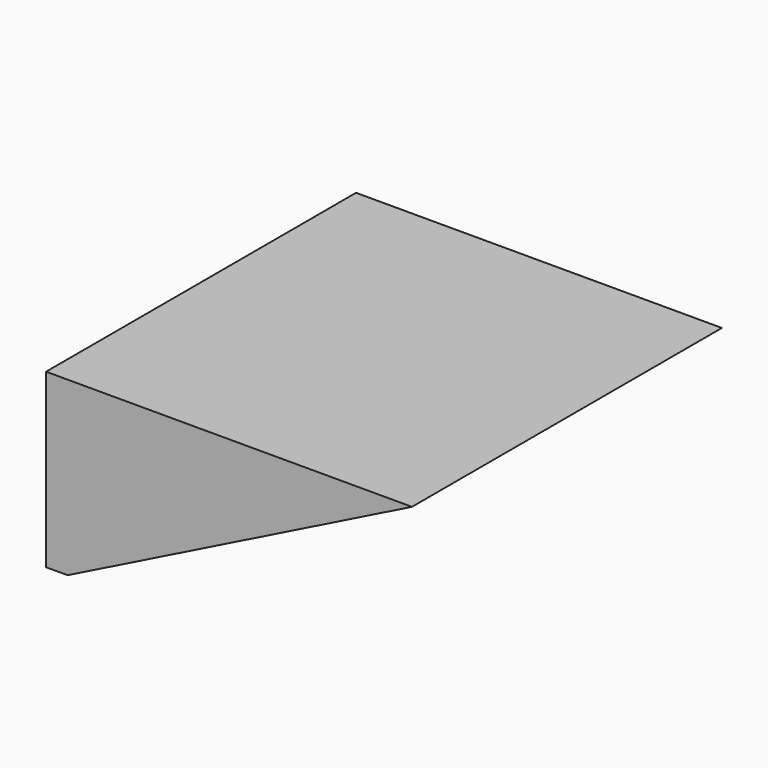
from build123d import *

# Parameters (mm, degrees)
F1_ANGLE      = 50
F3_DEPTH      = 25.4
F3_DEPTH_BACK = 25.4
F4_W          = 457.2
F4_H          = 203.2
F5_DEPTH      = 25.4
F7_DEPTH      = 406.4
F9_DEPTH      = 457.2


# Not quite as in the source:
# - ends of sketch curves that miss each other by under 0.0002 mm in the source are joined


with BuildPart() as f1:
    # F0 (on Top) → F1 (revolve)
    with BuildSketch(Plane.XY):
        with BuildLine():
            Line((-12.7, 12.7), (12.7, 12.7))
            ThreePointArc((12.7, 12.7), (0, 25.4), (-12.7, 12.7))
        make_face()
        with BuildLine():
            ThreePointArc((0, 0), (8.9802561211, 3.7197438789), (12.7, 12.7))
            Line((12.7, 12.7), (-12.7, 12.7))
            ThreePointArc((-12.7, 12.7), (-8.9802561211, 3.7197438789), (0, 0))
        make_face()
        with BuildLine():
            ThreePointArc((0, 0), (-8.9802561211, 3.7197438789), (-12.7, 12.7))
            Line((-12.7, 12.7), (-12.7, -12.7))
            ThreePointArc((-12.7, -12.7), (-8.9802561211, -3.7197438789), (0, 0))
        make_face()
        with BuildLine():
            Line((-12.7, -12.7), (12.7, -12.7))
            ThreePointArc((12.7, -12.7), (8.9802561211, -3.7197438789), (0, 0))
            ThreePointArc((0, 0), (-8.9802561211, -3.7197438789), (-12.7, -12.7))
        make_face()
        with BuildLine():
            ThreePointArc((-12.7, -12.7), (0, -25.4), (12.7, -12.7))
            Line((12.7, -12.7), (-12.7, -12.7))
        make_face()
        with BuildLine():
            Line((12.7, -12.7), (12.7, 12.7))
            ThreePointArc((12.7, 12.7), (8.9802561211, 3.7197438789), (0, 0))
            ThreePointArc((0, 0), (8.9802561211, -3.7197438789), (12.7, -12.7))
        make_face()
    revolve(axis=Axis((254, -3.8792621344, 0), (0, 1, 0)), revolution_arc=F1_ANGLE)

    # F2 (on Front) → F3 (cut, two sides)
    with BuildSketch(Plane.XZ) as f3_sk:
        Polygon((106.0351878405, 182.2580546141), (82.3100507259, 209.7299993038), (82.3100507259, 161.4786684513), align=None)
    extrude(amount=-F3_DEPTH, mode=Mode.SUBTRACT)
    extrude(f3_sk.sketch, amount=F3_DEPTH_BACK, mode=Mode.SUBTRACT)

    # F4 (on face) → F5 (join)
    with BuildSketch(Plane.YZ.offset(82.3100507259)):
        with Locations((0, 169.5530929186)):
            Rectangle(F4_W, F4_H)
        with BuildLine():
            Line((-12.7, 204.086871989), (12.7000006, 204.086871989))
            add(Edge.make_bspline(
                [(12.7000006, 204.086871989), (13.4690296338, 204.086871989), (14.2384453449, 204.0158750527), (14.9994460853, 203.8737558758), (15.7447177383, 203.6632719315), (16.4681309148, 203.3887393276), (17.1646524297, 203.0556697533), (18.2503222123, 202.4273420372), (18.6582844029, 202.1633436545), (19.0533520587, 201.8798852777), (19.4349362062, 201.5784262784), (19.8026309726, 201.2603920692), (20.1561814277, 200.9271325062), (20.9269905431, 200.1382361762), (21.3353938255, 199.6740027948), (21.7204670532, 199.1897069539), (22.0822142472, 198.6876735203), (22.420802674, 198.1700063327), (22.736519166, 197.6385568319), (23.250732617, 196.6851036415), (23.4589370134, 196.2683997588), (23.6544895384, 195.8454671817), (23.8375468192, 195.4169412733), (24.0082694094, 194.9834055779), (24.1668189946, 194.5453907771), (24.4233058083, 193.7717167394), (24.5264910507, 193.4378114469), (24.6229782806, 193.1018618849), (24.7128315819, 192.7640616927), (24.7961121661, 192.424594033), (24.8728783731, 192.0836315915), (25.1207544658, 190.876832951), (25.2571036638, 190.0039240497), (25.3531616976, 189.1251020116), (25.4096294667, 188.2427019804), (25.4270499712, 187.3589101884), (25.4057980417, 186.4757661893), (25.2856985057, 184.7074291559), (25.1862372229, 183.8224674602), (25.0477555884, 182.9421748337), (24.8701470857, 182.0686660516), (24.6531262016, 181.2042555644), (24.396196314, 180.3514681207), (23.98936689, 179.2056925756), (23.8747515893, 178.9002604218), (23.7546244835, 178.5969213548), (23.628943781, 178.2958298606), (23.4976641834, 177.9971515263), (23.3607368855, 177.7010630394), (23.0340408205, 177.0292176497), (22.8404825612, 176.6553180497), (22.6373184094, 176.286450794), (22.4244302808, 175.923064433), (22.2016988546, 175.5656585526), (21.9690040336, 175.2147836652), (21.4216371496, 174.439784246), (21.1012037916, 174.0197923426), (20.7646717024, 173.6122217846), (20.411845386, 173.2184579323), (20.0426129089, 172.8400922025), (19.6569713302, 172.4788991587), (18.9525917336, 171.8793804305), (18.6409356563, 171.6327871636), (18.3201611387, 171.3978713881), (17.9904282668, 171.175545954), (17.6519935165, 170.9667789735), (17.3052290423, 170.7725645788), (16.3872564507, 170.30998109), (15.8037606781, 170.0651084693), (15.202749403, 169.8635860217), (14.5874722629, 169.7092428977), (13.9619040353, 169.6051183146), (13.3308265381, 169.5530929186), (12.7, 169.5530929186)],
                knots=[0.5057352072, 0.5057352072, 0.5057352072, 0.5057352072, 0.5057352072, 0.5057352072, 0.5057352072, 0.5057352072, 0.6195246246, 0.6195246246, 0.6195246246, 0.6195246246, 0.6195246246, 0.6195246246, 0.691331529, 0.691331529, 0.691331529, 0.691331529, 0.691331529, 0.691331529, 0.7826631285, 0.7826631285, 0.7826631285, 0.7826631285, 0.7826631285, 0.7826631285, 0.8515046919, 0.8515046919, 0.8515046919, 0.8515046919, 0.8515046919, 0.8515046919, 0.9031583009, 0.9031583009, 0.9031583009, 0.9031583009, 0.9031583009, 0.9031583009, 1.0336151594, 1.0336151594, 1.0336151594, 1.0336151594, 1.0336151594, 1.0336151594, 1.1651272693, 1.1651272693, 1.1651272693, 1.1651272693, 1.1651272693, 1.1651272693, 1.2133438014, 1.2133438014, 1.2133438014, 1.2133438014, 1.2133438014, 1.2133438014, 1.275570012, 1.275570012, 1.275570012, 1.275570012, 1.275570012, 1.275570012, 1.3536385506, 1.3536385506, 1.3536385506, 1.3536385506, 1.3536385506, 1.3536385506, 1.412388273, 1.412388273, 1.412388273, 1.412388273, 1.412388273, 1.412388273, 1.5057352072, 1.5057352072, 1.5057352072, 1.5057352072, 1.5057352072, 1.5057352072, 1.5057352072, 1.5057352072], degree=7))
            Line((12.7, 169.5530929186), (-12.7000006, 169.5530929186))
            add(Edge.make_bspline(
                [(-12.7, 204.086871989), (-13.4706419927, 204.086871989), (-14.2416727155, 204.0155770292), (-15.0042333997, 203.8728607028), (-15.750966819, 203.6615047617), (-16.4757112201, 203.385859421), (-17.1734108274, 203.0514773721), (-18.2599454854, 202.421209965), (-18.6677421137, 202.1567547593), (-19.0626276136, 201.8728554308), (-19.4440153557, 201.5709719561), (-19.8115015564, 201.2525298833), (-20.1648331318, 200.9188788331), (-20.9351284745, 200.129125636), (-21.3432310697, 199.664436441), (-21.7279921591, 199.179709209), (-22.0894180876, 198.677267534), (-22.4276778241, 198.1592138164), (-22.7430593956, 197.6273980388), (-23.2566674815, 196.6733514115), (-23.4646047683, 196.2564127529), (-23.659888404, 195.8332560761), (-23.8426752316, 195.4045161634), (-24.0131259335, 194.9707760325), (-24.1714022488, 194.5325659004), (-24.4274032953, 193.7585803928), (-24.5303772724, 193.4245553586), (-24.626653065, 193.0884909648), (-24.7162947319, 192.7505806742), (-24.7993634474, 192.4110074931), (-24.8759175013, 192.0699439709), (-25.1230295402, 190.8628768117), (-25.2588319682, 189.9898251152), (-25.3543467105, 189.1108867647), (-25.4102732079, 188.2283952031), (-25.4271528417, 187.3445356956), (-25.4053586427, 186.4613475677), (-25.2841715299, 184.6930901591), (-25.184175573, 183.8082519745), (-25.0451643421, 182.9281062846), (-24.8670292224, 182.0547683599), (-24.6494826959, 181.1905540646), (-24.39202618, 180.337990515), (-23.9844834065, 179.1925931098), (-23.8696850934, 178.8872878707), (-23.7493755543, 178.584079685), (-23.6235129254, 178.2831232001), (-23.4920518465, 177.984584189), (-23.3549434604, 177.6886395502), (-23.0278434233, 177.0171551156), (-22.8340635577, 176.6434752959), (-22.630679354, 176.274835687), (-22.4175727111, 175.9116853585), (-22.1946243635, 175.5545244929), (-21.9617143535, 175.2039042681), (-21.413881263, 174.4295229159), (-21.0931995505, 174.009899279), (-20.7564242688, 173.6027135171), (-20.4033607941, 173.2093524612), (-20.0338985268, 172.8314090197), (-19.6480364418, 172.4706591125), (-18.9432894603, 171.8719538781), (-18.6314812112, 171.6257215316), (-18.3105623463, 171.3911796656), (-17.9806943678, 171.1692413992), (-17.6421353749, 170.9608748132), (-17.2952593711, 170.7670736149), (-16.3783249615, 170.3062381426), (-15.7960954678, 170.0625416452), (-15.196471078, 169.8620129232), (-14.5826838746, 169.7084467911), (-13.9586833556, 169.6048532006), (-13.3292171931, 169.5530929186), (-12.7000006, 169.5530929186)],
                knots=[0, 0, 0, 0, 0, 0, 0, 0, 0.1140276778, 0.1140276778, 0.1140276778, 0.1140276778, 0.1140276778, 0.1140276778, 0.1858507541, 0.1858507541, 0.1858507541, 0.1858507541, 0.1858507541, 0.1858507541, 0.2772036221, 0.2772036221, 0.2772036221, 0.2772036221, 0.2772036221, 0.2772036221, 0.3460585734, 0.3460585734, 0.3460585734, 0.3460585734, 0.3460585734, 0.3460585734, 0.3977198641, 0.3977198641, 0.3977198641, 0.3977198641, 0.3977198641, 0.3977198641, 0.5281851685, 0.5281851685, 0.5281851685, 0.5281851685, 0.5281851685, 0.5281851685, 0.6596880543, 0.6596880543, 0.6596880543, 0.6596880543, 0.6596880543, 0.6596880543, 0.7078965646, 0.7078965646, 0.7078965646, 0.7078965646, 0.7078965646, 0.7078965646, 0.7701090416, 0.7701090416, 0.7701090416, 0.7701090416, 0.7701090416, 0.7701090416, 0.8481566341, 0.8481566341, 0.8481566341, 0.8481566341, 0.8481566341, 0.8481566341, 0.906890942, 0.906890942, 0.906890942, 0.906890942, 0.906890942, 0.906890942, 1, 1, 1, 1, 1, 1, 1, 1], degree=7))
        make_face(mode=Mode.SUBTRACT)
        with BuildLine():
            add(Edge.make_bspline(
                [(12.7, 204.086871989), (13.4690296338, 204.086871989), (14.2384453449, 204.0158750527), (14.9994460853, 203.8737558758), (15.7447177383, 203.6632719315), (16.4681309148, 203.3887393276), (17.1646524297, 203.0556697533), (18.2503222123, 202.4273420372), (18.6582844029, 202.1633436545), (19.0533520587, 201.8798852777), (19.4349362062, 201.5784262784), (19.8026309726, 201.2603920692), (20.1561814277, 200.9271325062), (20.9269905431, 200.1382361762), (21.3353938255, 199.6740027948), (21.7204670532, 199.1897069539), (22.0822142472, 198.6876735203), (22.420802674, 198.1700063327), (22.736519166, 197.6385568319), (23.250732617, 196.6851036415), (23.4589370134, 196.2683997588), (23.6544895384, 195.8454671817), (23.8375468192, 195.4169412733), (24.0082694094, 194.9834055779), (24.1668189946, 194.5453907771), (24.4233058083, 193.7717167394), (24.5264910507, 193.4378114469), (24.6229782806, 193.1018618849), (24.7128315819, 192.7640616927), (24.7961121661, 192.424594033), (24.8728783731, 192.0836315915), (25.1207544658, 190.876832951), (25.2571036638, 190.0039240497), (25.3531616976, 189.1251020116), (25.4096294667, 188.2427019804), (25.4270499712, 187.3589101884), (25.4057980417, 186.4757661893), (25.2856985057, 184.7074291559), (25.1862372229, 183.8224674602), (25.0477555884, 182.9421748337), (24.8701470857, 182.0686660516), (24.6531262016, 181.2042555644), (24.396196314, 180.3514681207), (23.98936689, 179.2056925756), (23.8747515893, 178.9002604218), (23.7546244835, 178.5969213548), (23.628943781, 178.2958298606), (23.4976641834, 177.9971515263), (23.3607368855, 177.7010630394), (23.0340408205, 177.0292176497), (22.8404825612, 176.6553180497), (22.6373184094, 176.286450794), (22.4244302808, 175.923064433), (22.2016988546, 175.5656585526), (21.9690040336, 175.2147836652), (21.4216371496, 174.439784246), (21.1012037916, 174.0197923426), (20.7646717024, 173.6122217846), (20.411845386, 173.2184579323), (20.0426129089, 172.8400922025), (19.6569713302, 172.4788991587), (18.9525917336, 171.8793804305), (18.6409356563, 171.6327871636), (18.3201611387, 171.3978713881), (17.9904282668, 171.175545954), (17.6519935165, 170.9667789735), (17.3052290423, 170.7725645788), (16.3872564507, 170.30998109), (15.8037606781, 170.0651084693), (15.202749403, 169.8635860217), (14.5874722629, 169.7092428977), (13.9619040353, 169.6051183146), (13.3308265381, 169.5530929186), (12.7, 169.5530929186)],
                knots=[0.5057352072, 0.5057352072, 0.5057352072, 0.5057352072, 0.5057352072, 0.5057352072, 0.5057352072, 0.5057352072, 0.6195246246, 0.6195246246, 0.6195246246, 0.6195246246, 0.6195246246, 0.6195246246, 0.691331529, 0.691331529, 0.691331529, 0.691331529, 0.691331529, 0.691331529, 0.7826631285, 0.7826631285, 0.7826631285, 0.7826631285, 0.7826631285, 0.7826631285, 0.8515046919, 0.8515046919, 0.8515046919, 0.8515046919, 0.8515046919, 0.8515046919, 0.9031583009, 0.9031583009, 0.9031583009, 0.9031583009, 0.9031583009, 0.9031583009, 1.0336151594, 1.0336151594, 1.0336151594, 1.0336151594, 1.0336151594, 1.0336151594, 1.1651272693, 1.1651272693, 1.1651272693, 1.1651272693, 1.1651272693, 1.1651272693, 1.2133438014, 1.2133438014, 1.2133438014, 1.2133438014, 1.2133438014, 1.2133438014, 1.275570012, 1.275570012, 1.275570012, 1.275570012, 1.275570012, 1.275570012, 1.3536385506, 1.3536385506, 1.3536385506, 1.3536385506, 1.3536385506, 1.3536385506, 1.412388273, 1.412388273, 1.412388273, 1.412388273, 1.412388273, 1.412388273, 1.5057352072, 1.5057352072, 1.5057352072, 1.5057352072, 1.5057352072, 1.5057352072, 1.5057352072, 1.5057352072], degree=7))
            Line((12.7, 204.086871989), (-12.7, 204.086871989))
            add(Edge.make_bspline(
                [(-12.7, 204.086871989), (-13.4706419927, 204.086871989), (-14.2416727155, 204.0155770292), (-15.0042333997, 203.8728607028), (-15.750966819, 203.6615047617), (-16.4757112201, 203.385859421), (-17.1734108274, 203.0514773721), (-18.2599454854, 202.421209965), (-18.6677421137, 202.1567547593), (-19.0626276136, 201.8728554308), (-19.4440153557, 201.5709719561), (-19.8115015564, 201.2525298833), (-20.1648331318, 200.9188788331), (-20.9351284745, 200.129125636), (-21.3432310697, 199.664436441), (-21.7279921591, 199.179709209), (-22.0894180876, 198.677267534), (-22.4276778241, 198.1592138164), (-22.7430593956, 197.6273980388), (-23.2566674815, 196.6733514115), (-23.4646047683, 196.2564127529), (-23.659888404, 195.8332560761), (-23.8426752316, 195.4045161634), (-24.0131259335, 194.9707760325), (-24.1714022488, 194.5325659004), (-24.4274032953, 193.7585803928), (-24.5303772724, 193.4245553586), (-24.626653065, 193.0884909648), (-24.7162947319, 192.7505806742), (-24.7993634474, 192.4110074931), (-24.8759175013, 192.0699439709), (-25.1230295402, 190.8628768117), (-25.2588319682, 189.9898251152), (-25.3543467105, 189.1108867647), (-25.4102732079, 188.2283952031), (-25.4271528417, 187.3445356956), (-25.4053586427, 186.4613475677), (-25.2841715299, 184.6930901591), (-25.184175573, 183.8082519745), (-25.0451643421, 182.9281062846), (-24.8670292224, 182.0547683599), (-24.6494826959, 181.1905540646), (-24.39202618, 180.337990515), (-23.9844834065, 179.1925931098), (-23.8696850934, 178.8872878707), (-23.7493755543, 178.584079685), (-23.6235129254, 178.2831232001), (-23.4920518465, 177.984584189), (-23.3549434604, 177.6886395502), (-23.0278434233, 177.0171551156), (-22.8340635577, 176.6434752959), (-22.630679354, 176.274835687), (-22.4175727111, 175.9116853585), (-22.1946243635, 175.5545244929), (-21.9617143535, 175.2039042681), (-21.413881263, 174.4295229159), (-21.0931995505, 174.009899279), (-20.7564242688, 173.6027135171), (-20.4033607941, 173.2093524612), (-20.0338985268, 172.8314090197), (-19.6480364418, 172.4706591125), (-18.9432894603, 171.8719538781), (-18.6314812112, 171.6257215316), (-18.3105623463, 171.3911796656), (-17.9806943678, 171.1692413992), (-17.6421353749, 170.9608748132), (-17.2952593711, 170.7670736149), (-16.3783249615, 170.3062381426), (-15.7960954678, 170.0625416452), (-15.196471078, 169.8620129232), (-14.5826838746, 169.7084467911), (-13.9586833556, 169.6048532006), (-13.3292171931, 169.5530929186), (-12.7, 169.5530929186)],
                knots=[0, 0, 0, 0, 0, 0, 0, 0, 0.1140276778, 0.1140276778, 0.1140276778, 0.1140276778, 0.1140276778, 0.1140276778, 0.1858507541, 0.1858507541, 0.1858507541, 0.1858507541, 0.1858507541, 0.1858507541, 0.2772036221, 0.2772036221, 0.2772036221, 0.2772036221, 0.2772036221, 0.2772036221, 0.3460585734, 0.3460585734, 0.3460585734, 0.3460585734, 0.3460585734, 0.3460585734, 0.3977198641, 0.3977198641, 0.3977198641, 0.3977198641, 0.3977198641, 0.3977198641, 0.5281851685, 0.5281851685, 0.5281851685, 0.5281851685, 0.5281851685, 0.5281851685, 0.6596880543, 0.6596880543, 0.6596880543, 0.6596880543, 0.6596880543, 0.6596880543, 0.7078965646, 0.7078965646, 0.7078965646, 0.7078965646, 0.7078965646, 0.7078965646, 0.7701090416, 0.7701090416, 0.7701090416, 0.7701090416, 0.7701090416, 0.7701090416, 0.8481566341, 0.8481566341, 0.8481566341, 0.8481566341, 0.8481566341, 0.8481566341, 0.906890942, 0.906890942, 0.906890942, 0.906890942, 0.906890942, 0.906890942, 1, 1, 1, 1, 1, 1, 1, 1], degree=7))
            Line((-12.7, 169.5530929186), (12.7, 169.5530929186))
        make_face()
    extrude(amount=F5_DEPTH)

    # F6 (on face) → F7 (join)
    with BuildSketch(Plane.YZ.offset(107.7100507259)):
        Polygon((-222.25, 67.9530929186), (-222.25, 264.8030929186), (222.25, 264.8030929186), (222.25, 67.9530929186), (228.6, 67.9530929186), (228.6, 271.1530929186), (-228.6, 271.1530929186), (-228.6, 67.9530929186), align=None)
    extrude(amount=F7_DEPTH)

    # F8 (on face) → F9 (cut)
    with BuildSketch(Plane.XZ.offset(228.6)):
        Polygon((514.1100507259, 271.1530929186), (107.7100507259, 67.9530929186), (514.1100507259, 67.9530929186), align=None)
    extrude(amount=-F9_DEPTH, mode=Mode.SUBTRACT)


solid = f1.part
